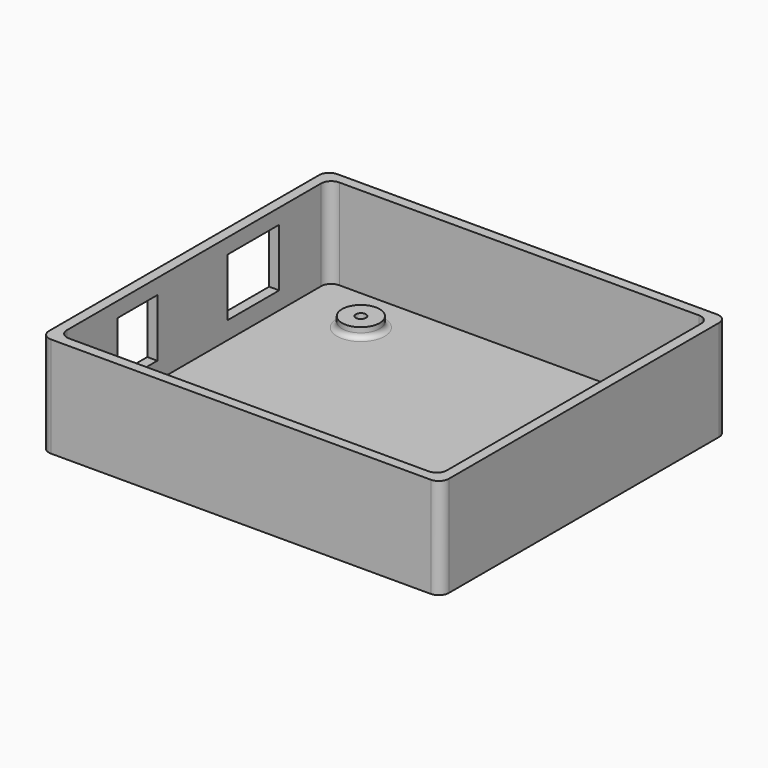
from build123d import *

# Parameters (mm, degrees)
F0_W      = 79.56
F0_H      = 71.2
F1_DEPTH  = 20
F3_R      = 2
F5_T      = 2
F6_R      = 2
F7_W      = 12.9
F7_H      = 11.5
F8_DEPTH  = 2
F9_W      = 9.9
F9_H      = 11.5
F10_DEPTH = 2
F11_R     = 3.75
F11_R_2   = 1
F12_DEPTH = 4
F13_R     = 1


# Not quite as in the source:
# - a shell that OpenCascade refuses in one call is made with other operations: the cavity is built on its own and cut out


with BuildPart() as f1:
    # F0 (on Top) → F1 (new body)
    with BuildSketch(Plane.XY):
        Rectangle(F0_W, F0_H)
    extrude(amount=F1_DEPTH)

    # F3
    f3_edges = [f1.edges().sort_by_distance(p)[0] for p in [
        (39.78, -35.6, 10),
        (39.78, 35.6, 10),
        (-39.78, 35.6, 10),
        (-39.78, -35.6, 10),
    ]]
    fillet(f3_edges, radius=F3_R)

    # F5: shell of thickness 2, made by hand


with BuildPart() as f5_core1:
    # F5_t2: copy of F1
    add(f1.part)

    # the walls: a layer under each face that stays
    f5_faces = [f5_core1.faces().sort_by_distance(p)[0] for p in [
        (0, 35.6, 10),
        (0, 0, 0),
        (39.78, 0, 10),
        (-39.78, 0, 10),
        (0, -35.6, 10),
    ]]
    thicken(f5_faces, amount=-F5_T, mode=Mode.SUBTRACT)


with BuildPart() as f1_1:
    add(f1.part)

    # what is left inside the walls is the cavity
    f5_cavity = [f5_core1.part.solids().sort_by_distance(p)[0] for p in [
        (0, -11.2, 2.02),
    ]]
    add(f5_cavity, mode=Mode.SUBTRACT)

    # F6
    f6_edges = [f1_1.edges().sort_by_distance(p)[0] for p in [
        (-37.78, 33.6, 11),
        (37.78, 33.6, 11),
        (-37.78, -33.6, 11),
        (37.78, -33.6, 11),
    ]]
    fillet(f6_edges, radius=F6_R)

    # F7 (on face) → F8 (cut)
    with BuildSketch(Plane(origin=(-39.78, 0, 0), x_dir=(0, -1, 0), z_dir=(-1, 0, 0))):
        with Locations((-14.72, 11.25)):
            Rectangle(F7_W, F7_H)
    extrude(amount=-F8_DEPTH, mode=Mode.SUBTRACT)

    # F9 (on face) → F10 (cut)
    with BuildSketch(Plane(origin=(-39.78, 0, 0), x_dir=(0, -1, 0), z_dir=(-1, 0, 0))):
        with Locations((14.08, 11.25)):
            Rectangle(F9_W, F9_H)
    extrude(amount=-F10_DEPTH, mode=Mode.SUBTRACT)

    # F11 (on Top) → F12 (join)
    with BuildSketch(Plane.XY):
        with Locations((-24.28, 24.6)):
            Circle(F11_R)
        with Locations((-24.28, 24.6)):
            Circle(F11_R_2, mode=Mode.SUBTRACT)
        with Locations((27.5, 9.88)):
            Circle(F11_R)
        with Locations((27.5, 9.88)):
            Circle(F11_R_2, mode=Mode.SUBTRACT)
        with Locations((-24.28, -21.6)):
            Circle(F11_R)
        with Locations((-24.28, -21.6)):
            Circle(F11_R_2, mode=Mode.SUBTRACT)
        with Locations((27.5, -16.62)):
            Circle(F11_R)
        with Locations((27.5, -16.62)):
            Circle(F11_R_2, mode=Mode.SUBTRACT)
    extrude(amount=F12_DEPTH)

    # F13
    f13_edges = [f1_1.edges().sort_by_distance(p)[0] for p in [
        (-28.03, 24.6, 2),
        (-28.03, -21.6, 2),
        (23.75, 9.88, 2),
        (23.75, -16.62, 2),
    ]]
    fillet(f13_edges, radius=F13_R)


solid = f1_1.part
